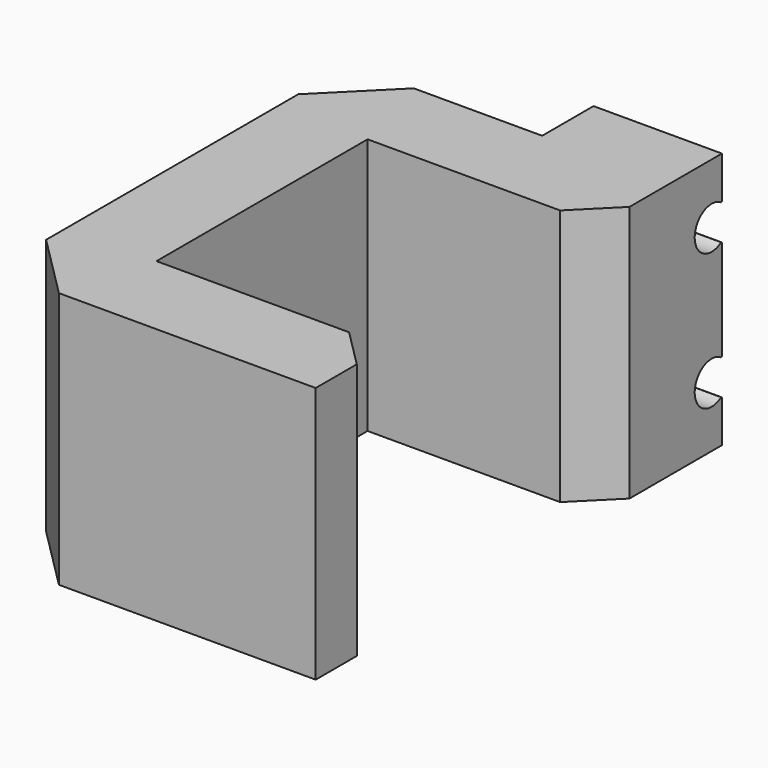
from build123d import *

# Parameters (mm, degrees)
F1_DEPTH    = 20
F3_DEPTH    = 10
F4_SIZE     = 3
F5_T1_DEPTH = 10.4919836734
F6_SIZE     = 5


# Not quite as in the source:
# - a fillet or chamfer that OpenCascade refuses, or shapes differently, is made with other operations: its cross-section is extruded or revolved along the edge and cut away or added


with BuildPart() as f1:
    # F0 (on Top) → F1 (new body)
    with BuildSketch(Plane.XY):
        Polygon((11, 17.275), (-14, 17.275), (-14, -17.275), (11, -17.275), (11, -10.275), (-7, -10.275), (-7, 10.275), (11, 10.275), align=None)
    extrude(amount=F1_DEPTH)

    # F2 (on face) → F3 (join)
    with BuildSketch(Plane.YZ.offset(11)):
        with BuildLine():
            ThreePointArc((22.275, 14), (19.625, 15.3124404748), (22.275, 16.6248809497))
            Line((22.275, 16.6248809497), (22.275, 20))
            Line((22.275, 20), (17.275, 20))
            Line((17.275, 20), (17.275, 0))
            Line((17.275, 0), (22.275, 0))
            Line((22.275, 0), (22.275, 3.3751190503))
            ThreePointArc((22.275, 3.3751190503), (19.625, 4.6875595252), (22.275, 6))
            Line((22.275, 6), (22.275, 14))
        make_face()
    extrude(amount=-F3_DEPTH)

    # F4
    f4_edges = [f1.edges().sort_by_distance(p)[0] for p in [
        (11, 10.275, 10),
        (11, -10.275, 10),
    ]]
    chamfer(f4_edges, length=F4_SIZE)

    # F5: chamfer of 0.1 on 4 edges, made by hand

    # F5_s2 → F5_t1 (cut)
    with BuildSketch(Plane.YZ.offset(0.7540081633)):
        with BuildLine():
            Line((22.2785318644, 16.7232142773), (22.1942442254, 16.6784020049))
            Line((22.1942442254, 16.6784020049), (22.193125709, 16.6767440179))
            ThreePointArc((22.193125709, 16.6767440179), (22.2348996139, 16.6520287441), (22.2737878788, 16.6232901127))
            Line((22.2737878788, 16.6232901127), (22.277, 16.6248809497))
            ThreePointArc((22.277, 16.6248809497), (22.277, 16.6740476135), (22.2805318644, 16.7232142773))
            Line((22.2805318644, 16.7232142773), (22.2785318644, 16.7232142773))
        make_face()
        with BuildLine():
            Line((22.1942442254, 13.9464789448), (22.2785318644, 13.9016666723))
            Line((22.2785318644, 13.9016666723), (22.2805318644, 13.9016666723))
            ThreePointArc((22.2805318644, 13.9016666723), (22.277, 13.9508333362), (22.277, 14))
            Line((22.277, 14), (22.2737878788, 14.0015908369))
            ThreePointArc((22.2737878788, 14.0015908369), (22.2348996139, 13.9728522055), (22.193125709, 13.9481369318))
            Line((22.193125709, 13.9481369318), (22.1942442254, 13.9464789448))
        make_face()
        with BuildLine():
            Line((22.2785318644, 6.0983333277), (22.1942442254, 6.0535210552))
            Line((22.1942442254, 6.0535210552), (22.193125709, 6.0518630682))
            ThreePointArc((22.193125709, 6.0518630682), (22.2348996139, 6.0271477945), (22.2737878788, 5.9984091631))
            Line((22.2737878788, 5.9984091631), (22.277, 6))
            ThreePointArc((22.277, 6), (22.277, 6.0491666638), (22.2805318644, 6.0983333277))
            Line((22.2805318644, 6.0983333277), (22.2785318644, 6.0983333277))
        make_face()
        with BuildLine():
            Line((22.2785318644, 3.2767857227), (22.1942442254, 3.3215979951))
            Line((22.1942442254, 3.3215979951), (22.193125709, 3.3232559821))
            ThreePointArc((22.193125709, 3.3232559821), (22.2348996139, 3.3479712559), (22.2737878788, 3.3767098873))
            Line((22.2737878788, 3.3767098873), (22.277, 3.3751190503))
            ThreePointArc((22.277, 3.3751190503), (22.277, 3.3259523865), (22.2805318644, 3.2767857227))
            Line((22.2805318644, 3.2767857227), (22.2785318644, 3.2767857227))
        make_face()
    extrude(amount=F5_T1_DEPTH, mode=Mode.SUBTRACT)

    # F6
    f6_edges = [f1.edges().sort_by_distance(p)[0] for p in [
        (-14, 17.275, 10),
        (-14, -17.275, 10),
    ]]
    chamfer(f6_edges, length=F6_SIZE)


solid = f1.part
